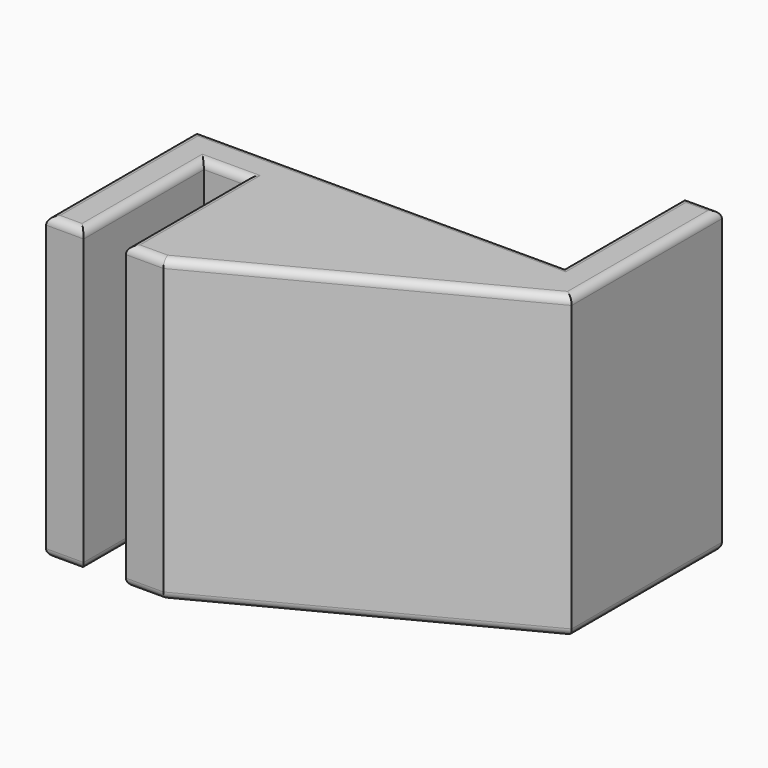
from build123d import *

# Parameters (mm, degrees)
F1_DEPTH     = 76.2
F2_R         = 2
F3_TEXT_SIZE = 8.7088824601
F4_DEPTH     = 0.5


# Not quite as in the source:
# - Text() gives the source's letters only with a copy of the font that has no kerning and outlines rounded to 1/6400 em; it was checked with that copy


with BuildPart() as f1:
    # F0 (on Top) → F1 (new body)
    with BuildSketch(Plane.XY):
        Polygon((-29.75, 9.525), (-29.75, -38.1), (-20.225, -38.1), (-20.225, 0), (-9.525, 0), (-9.525, -38.1), (0, -38.1), (0, 0), (73.025, 0), (73.025, 47.625), (63.5, 47.625), (63.5, 9.525), align=None)
        Polygon((0, -38.1), (73.025, 0), (0, 0), align=None)
    extrude(amount=F1_DEPTH)

    # F2
    f2_edges = [f1.edges().sort_by_distance(p)[0] for p in [
        (-29.75, -14.2875, 0),
        (-24.9875, -38.1, 0),
        (-20.225, -19.05, 0),
        (-14.875, 0, 0),
        (-9.525, -19.05, 0),
        (-4.7625, -38.1, 0),
        (36.5125, -19.05, 0),
        (73.025, 23.8125, 0),
        (68.2625, 47.625, 0),
        (63.5, 28.575, 0),
        (16.875, 9.525, 0),
        (-29.75, -14.2875, 76.2),
        (-24.9875, -38.1, 76.2),
        (-20.225, -19.05, 76.2),
        (-14.875, 0, 76.2),
        (-9.525, -19.05, 76.2),
        (-4.7625, -38.1, 76.2),
        (36.5125, -19.05, 76.2),
        (73.025, 23.8125, 76.2),
        (68.2625, 47.625, 76.2),
        (63.5, 28.575, 76.2),
        (16.875, 9.525, 76.2),
    ]]
    fillet(f2_edges, radius=F2_R)

    # F3 (on face) → F4 (cut)
    with BuildSketch(Plane(origin=(-29.75, 0, 0), x_dir=(0, -1, 0), z_dir=(-1, 0, 0))):
        with Locations(Location((28.1, 6.35), (0, 0, 90))):
            Text('printed3d.parts', F3_TEXT_SIZE, font='Open Sans', text_align=(TextAlign.LEFT, TextAlign.BOTTOM))
    extrude(amount=-F4_DEPTH, mode=Mode.SUBTRACT)


solid = f1.part
